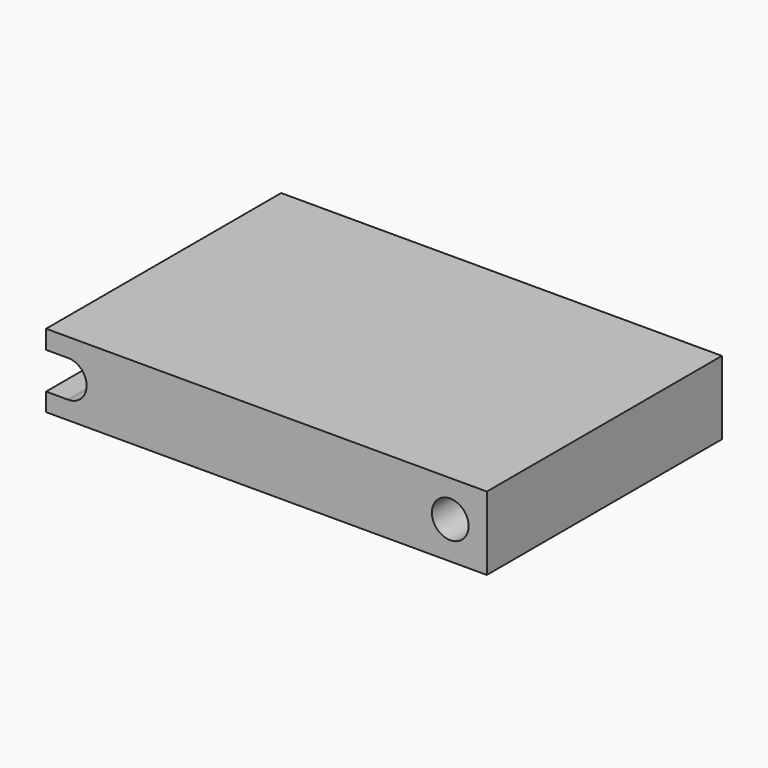
from build123d import *

# Parameters (mm, degrees)
F0_R     = 4.7625
F1_DEPTH = 76.2


# Not quite as in the source:
# - the program builds the solid bodies; features that only make, move or delete a surface that nothing else refers to are left out


with BuildPart() as f1:
    # F0 (on Front) → F1 (new body)
    with BuildSketch(Plane.XZ):
        with BuildLine():
            Line((-114.3, 0), (0, 0))
            Line((0, 0), (0, 19.05))
            Line((0, 19.05), (-114.3, 19.05))
            Line((-114.3, 19.05), (-114.3, 14.2229856587))
            Line((-114.3, 14.2229856587), (-108.7215644084, 14.2229856587))
            ThreePointArc((-108.7215644084, 14.2229856587), (-105.2435953967, 12.891306681), (-103.7874654915, 9.4635781261))
            ThreePointArc((-103.7874654915, 9.4635781261), (-105.1136603504, 6.1661225575), (-108.3536442745, 4.7051262529))
            ThreePointArc((-108.3536442745, 4.7051262529), (-108.5499654915, 4.7010781261), (-108.7462867086, 4.7051262529))
            Line((-108.7462867086, 4.7051262529), (-114.3, 4.7051262529))
            Line((-114.3, 4.7051262529), (-114.3, 0))
        make_face()
        with Locations((-9.4899654915, 9.609828106)):
            Circle(F0_R, mode=Mode.SUBTRACT)
    extrude(amount=F1_DEPTH)


solid = f1.part
